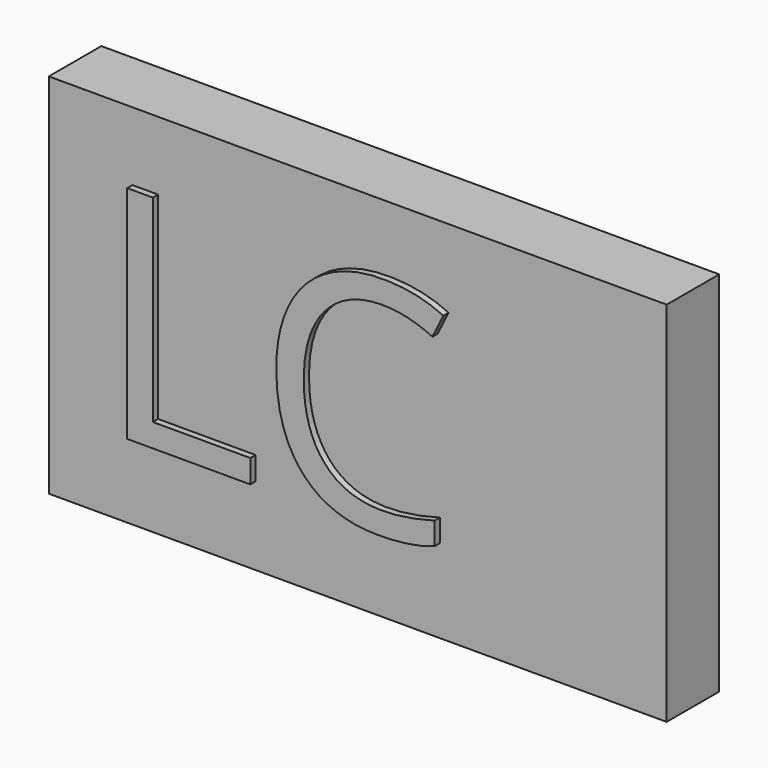
from build123d import *

# Parameters (mm, degrees)
F0_W         = 94.1131487489
F0_H         = 55.9516921639
F1_DEPTH     = 10
F2_TEXT_SIZE = 47.106079809
F3_DEPTH     = 1


# Not quite as in the source:
# - Text() gives the source's letters only with a copy of the font that has no kerning and outlines rounded to 1/6400 em; it was checked with that copy


with BuildPart() as f1:
    # F0 (on Front) → F1 (new body)
    with BuildSketch(Plane.XZ):
        with Locations((47.0565743744, 27.975846082)):
            Rectangle(F0_W, F0_H)
    extrude(amount=F1_DEPTH)

    # F2 (on face) → F3 (join)
    with BuildSketch(Plane.XZ.offset(10)):
        with Locations((8.1239640713, 11.8911927566)):
            Text('LC', F2_TEXT_SIZE, font='Open Sans', text_align=(TextAlign.LEFT, TextAlign.BOTTOM))
    extrude(amount=F3_DEPTH)


solid = f1.part
